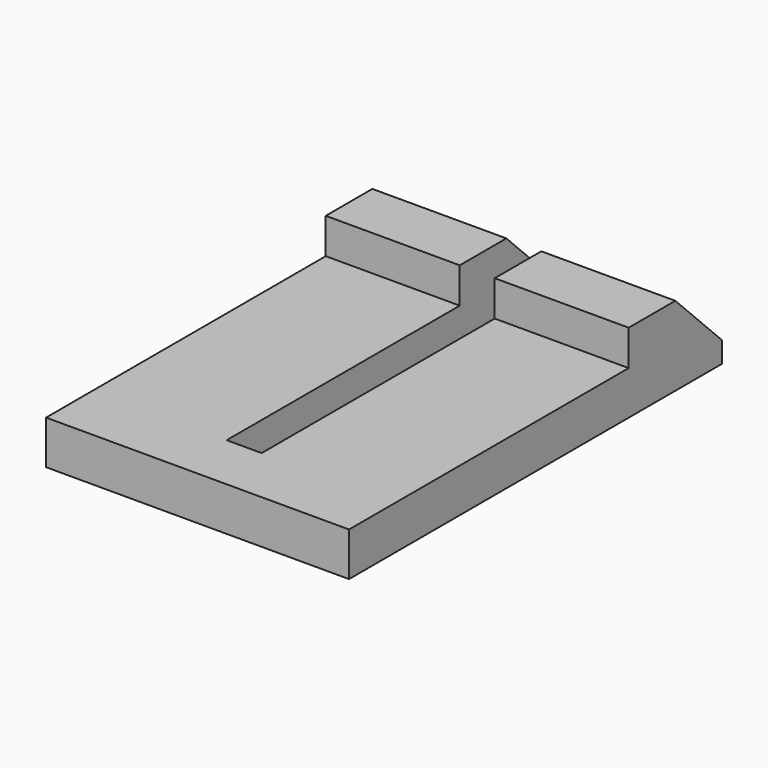
from build123d import *

# Parameters (mm, degrees)
F0_W     = 11.5
F0_H     = 25
F0_W_2   = 1.5
F0_H_2   = 5
F1_DEPTH = 3.75
F0_H_3   = 10
F2_DEPTH = 6.8
F3_SIZE  = 5


with BuildPart() as f1:
    # F0 (on Top) → F1 (new body)
    with BuildSketch(Plane.XY):
        with Locations((-7.25, 17.5)):
            Rectangle(F0_W, F0_H)
        Polygon((1.5, 30), (1.5, 5), (13, 4.9315184347), (13, 30), align=None)
        Polygon((1.5, 5), (1.5, 0), (13, 0), (13, 4.9315184347), align=None)
        with Locations((0.75, 2.5)):
            Rectangle(F0_W_2, F0_H_2)
        with Locations((-0.75, 2.5)):
            Rectangle(F0_W_2, F0_H_2)
        with Locations((-7.25, 2.5)):
            Rectangle(F0_W, F0_H_2)
    extrude(amount=F1_DEPTH)

    # F0 (on Top) → F2 (join)
    with BuildSketch(Plane.XY):
        with Locations((-7.25, 35)):
            Rectangle(F0_W, F0_H_3)
        with Locations((7.25, 35)):
            Rectangle(F0_W, F0_H_3)
    extrude(amount=F2_DEPTH)

    # F3
    f3_edges = [f1.edges().sort_by_distance(p)[0] for p in [
        (-7.25, 40, 6.8),
        (7.25, 40, 6.8),
    ]]
    chamfer(f3_edges, length=F3_SIZE)


solid = f1.part
